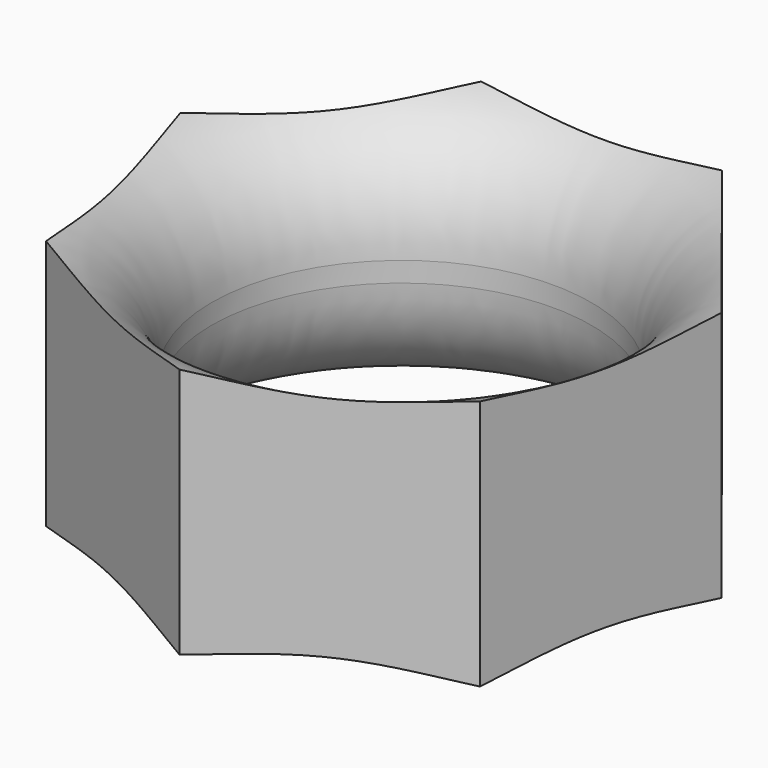
from build123d import *

# Parameters (mm, degrees)
F0_R     = 9.5
F1_DEPTH = 13


# Not quite as in the source:
# - a fillet or chamfer that OpenCascade refuses, or shapes differently, is made with other operations: its cross-section is extruded or revolved along the edge and cut away or added


with BuildPart() as f1:
    # F0 (on Top) → F1 (new body)
    with BuildSketch(Plane.XY):
        Polygon((6.024763409, 12.5105501281), (-6.024763409, 12.5105501281), (-13.5375204973, 3.0898507129), (-10.856248536, -8.6575693106), (0, -13.885663061), (10.856248536, -8.6575693106), (13.5375204973, 3.0898507129), align=None)
        Circle(F0_R, mode=Mode.SUBTRACT)
    extrude(amount=F1_DEPTH)

    # F2: fillet of radius 6 on 3 edges, made by hand

    # F2_s1 → F2_t2 (revolve, cut)
    with BuildSketch(Plane.XZ):
        with BuildLine():
            ThreePointArc((9.5, 6), (11.2573593129, 1.7573593129), (15.5, 0))
            Line((15.5, 0), (9.5, 0))
            Line((9.5, 0), (9.5, 6))
        make_face()
    revolve(axis=Axis((0, 0, 0), (0, 0, 1)), mode=Mode.SUBTRACT)

    # F2_s3 → F2_t4 (revolve, cut)
    with BuildSketch(Plane.XZ):
        with BuildLine():
            ThreePointArc((9.5, 7), (11.2573593129, 11.2426406871), (15.5, 13))
            Line((15.5, 13), (9.5, 13))
            Line((9.5, 13), (9.5, 7))
        make_face()
    revolve(axis=Axis((0, 0, 13), (0, 0, 1)), mode=Mode.SUBTRACT)


solid = f1.part
